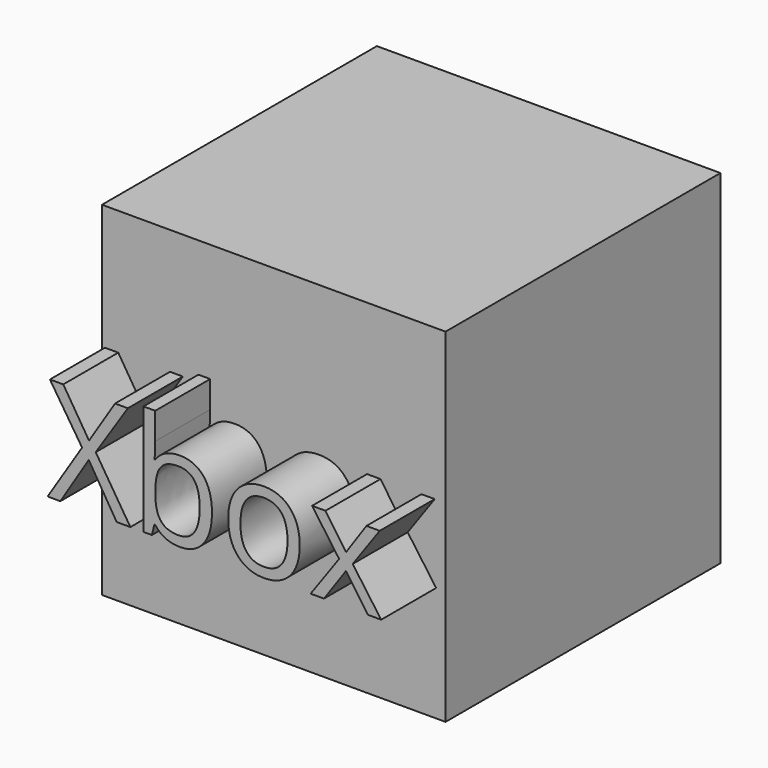
from build123d import *

# Parameters (mm, degrees)
F0_W         = 25.4
F0_H         = 25.4
F1_DEPTH     = 25.4
F2_TEXT_SIZE = 10.7499008068
F3_DEPTH     = 5.08


# Not quite as in the source:
# - Text() gives the source's letters only with a copy of the font that has no kerning and outlines rounded to 1/6400 em; it was checked with that copy


with BuildPart() as f1:
    # F0 (on Front) → F1 (new body)
    with BuildSketch(Plane.XZ):
        with Locations((12.7, 12.7)):
            Rectangle(F0_W, F0_H)
    extrude(amount=F1_DEPTH)

    # F2 (on face) → F3 (join)
    with BuildSketch(Plane.XZ.offset(25.4)):
        with Locations((0, 8.4898468628)):
            Text('Xbox', F2_TEXT_SIZE, font='Open Sans', text_align=(TextAlign.LEFT, TextAlign.BOTTOM))
    extrude(amount=F3_DEPTH)


solid = f1.part
